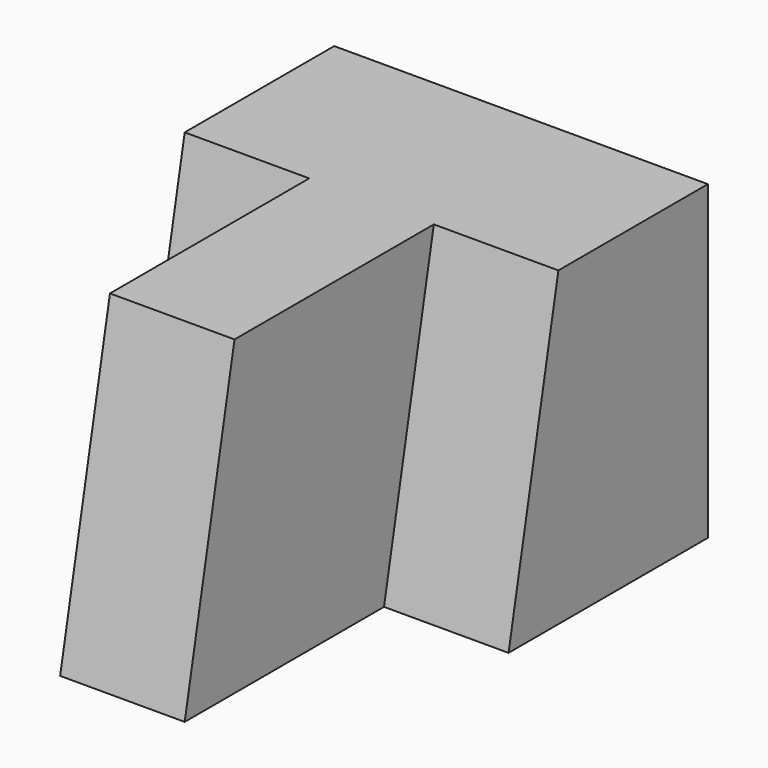
from build123d import *

# Parameters (mm, degrees)
F0_W      = 38.1
F0_H      = 31.75
F1_DEPTH  = 44.45
F2_W      = 12.7
F2_H      = 31.75
F3_DEPTH  = 19.05
F5_DEPTH  = 12.7
F7_DEPTH  = 12.7
F8_DEPTH  = 6.35
F10_DEPTH = 25.4


# Not quite as in the source:
# - a feature names something its author has since deleted; it is built from what else it names


with BuildPart() as f1:
    # F0 (on Front) → F1 (new body)
    with BuildSketch(Plane.XZ):
        with Locations((19.05, 15.875)):
            Rectangle(F0_W, F0_H)
    extrude(amount=F1_DEPTH)

    # F2 (on face) → F3 (cut)
    with BuildSketch(Plane.XZ.offset(44.45)):
        with Locations((31.75, 15.875)):
            Rectangle(F2_W, F2_H)
        with Locations((6.35, 15.875)):
            Rectangle(F2_W, F2_H)
    extrude(amount=-F3_DEPTH, mode=Mode.SUBTRACT)

    # F4 (on face) → F5 (cut)
    with BuildSketch(Plane.YZ.offset(38.1)):
        Polygon((-25.4, 0), (-19.05, 31.75), (-25.4, 31.75), align=None)
    extrude(amount=-F5_DEPTH, mode=Mode.SUBTRACT)

    # F6 (on face) → F7 (cut)
    with BuildSketch(Plane(origin=(0, 0, 0), x_dir=(0, -1, 0), z_dir=(-1, 0, 0))):
        Polygon((25.4, 0), (25.4, 31.75), (19.05, 31.75), align=None)
    extrude(amount=-F7_DEPTH, mode=Mode.SUBTRACT)

    # F8 (add): a face of the model
    f8_faces = [f1.faces().sort_by_distance(p)[0] for p in [
        (19.05, -44.45, 15.875),
    ]]
    extrude(f8_faces, amount=F8_DEPTH)

    # F9 (on face) → F10 (cut)
    with BuildSketch(Plane.YZ.offset(25.4)):
        Polygon((-50.8, 0), (-44.45, 31.75), (-50.8, 31.75), align=None)
    extrude(amount=-F10_DEPTH, mode=Mode.SUBTRACT)


solid = f1.part
